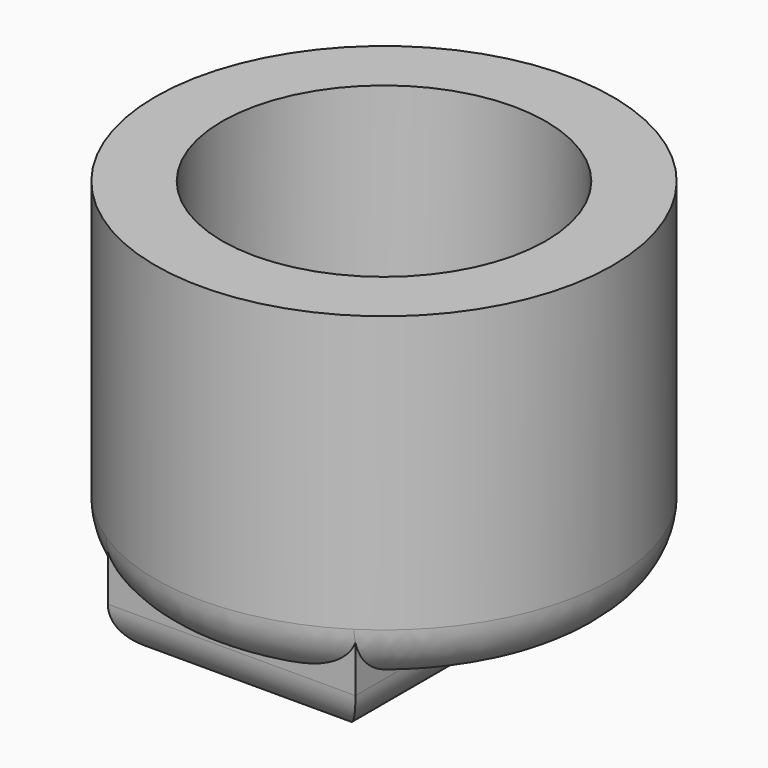
from build123d import *

# Parameters (mm, degrees)
F1_DEPTH = 3
F2_R     = 4.25
F3_DEPTH = 7
F4_T     = 1.75
F6_R     = 1.2


# Not quite as in the source:
# - a fillet or chamfer that OpenCascade refuses, or shapes differently, is made with other operations: its cross-section is extruded or revolved along the edge and cut away or added


with BuildPart() as f1:
    # F0 (on Right) → F1 (new body)
    with BuildSketch(Plane.YZ):
        Polygon((-3.25, -1.5), (3.25, -1.5), (3.25, 1.5), (0, 1.5), (-3.25, 1.5), align=None)
    extrude(amount=F1_DEPTH)

    # F2 (on face) → F3 (join)
    with BuildSketch(Plane.XY.offset(1.5)):
        with Locations((1.5, 0)):
            Circle(F2_R)
    extrude(amount=F3_DEPTH)

    # F4
    f4_openings = [f1.faces().sort_by_distance(p)[0] for p in [
        (1.5, 0, -1.5),
        (1.5, 0, 8.5),
    ]]
    offset(amount=F4_T, openings=f4_openings, kind=Kind.INTERSECTION)

    # F5: fillet of radius 1.5 on 1 edges, made by hand


with BuildPart() as f5_tool2:
    # F5_s3 → F5_t4 (revolve)
    with BuildSketch(Plane.XZ):
        with BuildLine():
            ThreePointArc((7.5, 1.25), (7.0606601718, 0.1893398282), (6, -0.25))
            Line((6, -0.25), (7.5, -0.25))
            Line((7.5, -0.25), (7.5, 1.25))
        make_face()
    revolve(axis=Axis((1.5, 0, -0.25), (0, 0, -1)))

    split(bisect_by=Plane.YZ.offset(4.75), keep=Keep.TOP)


with BuildPart() as f1_1:
    add(f1.part)

    # F5_t1: cut F5_tool2
    add(f5_tool2.part, mode=Mode.SUBTRACT)


with BuildPart() as f5_tool7:
    # F5_s8 → F5_t9 (revolve)
    with BuildSketch(Plane.XZ):
        with BuildLine():
            ThreePointArc((7.5, 1.25), (7.0606601718, 0.1893398282), (6, -0.25))
            Line((6, -0.25), (7.5, -0.25))
            Line((7.5, -0.25), (7.5, 1.25))
        make_face()
    revolve(axis=Axis((1.5, 0, -0.25), (0, 0, -1)))

    split(bisect_by=Plane.YZ.offset(-1.75), keep=Keep.BOTTOM)


with BuildPart() as f1_2:
    add(f1_1.part)

    # F5_t6: cut F5_tool7
    add(f5_tool7.part, mode=Mode.SUBTRACT)


with BuildPart() as f5_tool12:
    # F5_s13 → F5_t14 (revolve)
    with BuildSketch(Plane.XZ):
        with BuildLine():
            ThreePointArc((7.5, 1.25), (7.0606601718, 0.1893398282), (6, -0.25))
            Line((6, -0.25), (7.5, -0.25))
            Line((7.5, -0.25), (7.5, 1.25))
        make_face()
    revolve(axis=Axis((1.5, 0, -0.25), (0, 0, -1)))

    split(bisect_by=Plane.XZ.offset(5), keep=Keep.TOP)


with BuildPart() as f1_3:
    add(f1_2.part)

    # F5_t11: cut F5_tool12
    add(f5_tool12.part, mode=Mode.SUBTRACT)


with BuildPart() as f5_tool17:
    # F5_s18 → F5_t19 (revolve)
    with BuildSketch(Plane.XZ):
        with BuildLine():
            ThreePointArc((7.5, 1.25), (7.0606601718, 0.1893398282), (6, -0.25))
            Line((6, -0.25), (7.5, -0.25))
            Line((7.5, -0.25), (7.5, 1.25))
        make_face()
    revolve(axis=Axis((1.5, 0, -0.25), (0, 0, -1)))

    split(bisect_by=Plane.XZ.offset(-5), keep=Keep.BOTTOM)


with BuildPart() as f1_4:
    add(f1_3.part)

    # F5_t16: cut F5_tool17
    add(f5_tool17.part, mode=Mode.SUBTRACT)

    # F6
    f6_edges = [f1_4.edges().sort_by_distance(p)[0] for p in [
        (1.5, 5, -1.5),
        (4.75, 0, -1.5),
        (1.5, -5, -1.5),
        (-1.75, 0, -1.5),
    ]]
    fillet(f6_edges, radius=F6_R)


solid = f1_4.part
